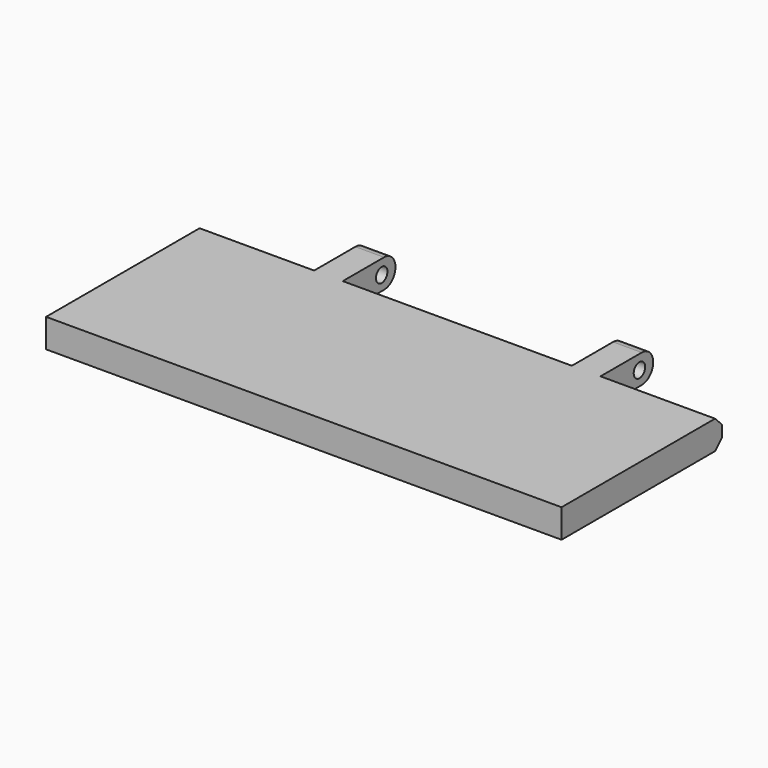
from build123d import *

# Parameters (mm, degrees)
F0_W     = 180
F0_H     = 70
F1_DEPTH = 10
F3_W     = 10
F3_H     = 10
F4_DEPTH = 20
F5_R     = 2.5
F6_DEPTH = 140.001
F7_R     = 4.99999
F8_SIZE  = 3


# Not quite as in the source:
# - a fillet or chamfer is up to 0.001 mm smaller than in the source, because OpenCascade refuses the exact size


with BuildPart() as f1:
    # F0 (on Top) → F1 (new body)
    with BuildSketch(Plane.XY):
        with Locations((90, 35)):
            Rectangle(F0_W, F0_H)
    extrude(amount=F1_DEPTH)

    # F3 (on face) → F4 (join)
    with BuildSketch(Plane(origin=(0, 70, 0), x_dir=(-1, 0, 0), z_dir=(0, 1, 0))):
        with Locations((-135, 5)):
            Rectangle(F3_W, F3_H)
        with Locations((-45, 5)):
            Rectangle(F3_W, F3_H)
    extrude(amount=F4_DEPTH)

    # F5 (on face) → F6 (cut, through all)
    with BuildSketch(Plane(origin=(40, 0, 0), x_dir=(0, -1, 0), z_dir=(-1, 0, 0))):
        with Locations((-84, 5)):
            Circle(F5_R)
    extrude(amount=-F6_DEPTH, mode=Mode.SUBTRACT)

    # F7 (radius 5 in the source; OpenCascade refuses exactly that, so slightly less here)
    f7_edges = [f1.edges().sort_by_distance(p)[0] for p in [
        (135, 90, 10),
        (135, 90, 0),
        (45, 90, 0),
        (45, 90, 10),
    ]]
    fillet(f7_edges, radius=F7_R)

    # F8
    f8_edges = [f1.edges().sort_by_distance(p)[0] for p in [
        (90, 70, 10),
        (20, 70, 10),
        (160, 70, 10),
        (160, 70, 0),
        (90, 70, 0),
        (20, 70, 0),
    ]]
    chamfer(f8_edges, length=F8_SIZE)


solid = f1.part
